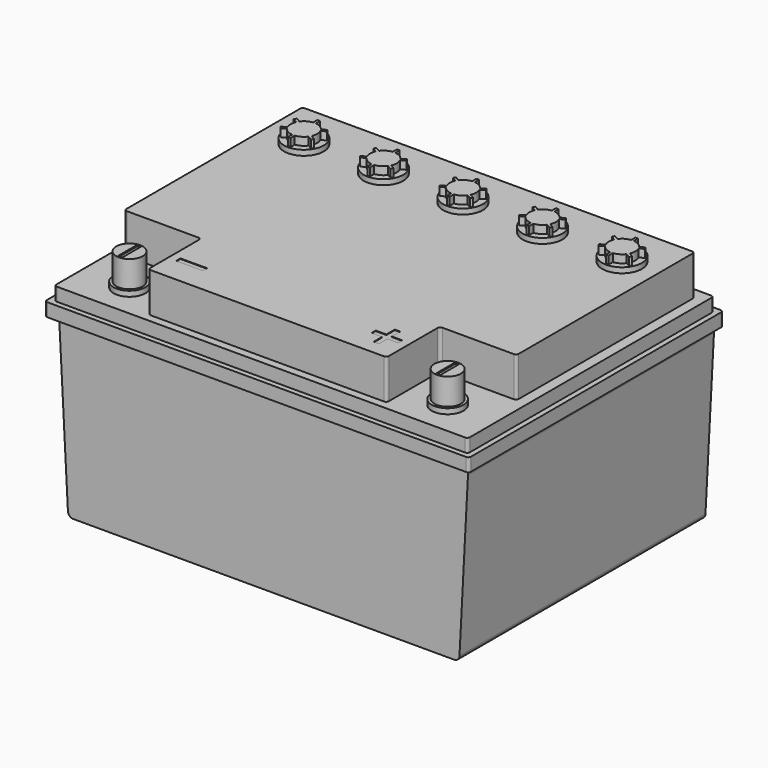
from build123d import *

# Parameters (mm, degrees)
F0_W      = 160
F0_H      = 120
F1_DEPTH  = 5
F2_W      = 156
F2_H      = 116
F3_DEPTH  = 5
F5_DEPTH  = 15
F6_R      = 6
F7_DEPTH  = 2
F8_R      = 5
F9_DEPTH  = 10
F10_R     = 7.5
F11_DEPTH = 2
F13_DEPTH = 3
F14_W     = 1.6
F14_H     = 9.2
F15_DEPTH = 0.5
F16_R     = 1
F17_W     = 10
F17_H     = 1
F18_DEPTH = 0.2
F20_DEPTH = 116


# Not quite as in the source:
# - a feature names something its author has since deleted; it is built from what else it names


with BuildPart() as f1:
    # F0 (on Top) → F1 (new body)
    with BuildSketch(Plane.XY):
        Rectangle(F0_W, F0_H)
    extrude(amount=F1_DEPTH)

    # F2 (on face) → F3 (join)
    with BuildSketch(Plane.XY.offset(5)):
        Rectangle(F2_W, F2_H)
    extrude(amount=F3_DEPTH)

    # F4 (on face) → F5 (join)
    with BuildSketch(Plane.XY.offset(10)):
        Polygon((74, 54), (-74, 54), (-74, -30), (-45, -30), (-45, -55), (45, -55), (45, -30), (74, -30), align=None)
    extrude(amount=F5_DEPTH)

    # F6 (on face) → F7 (join)
    with BuildSketch(Plane.XY.offset(10)):
        with Locations((-60, -45)):
            Circle(F6_R)
        with Locations((60, -45)):
            Circle(F6_R)
    extrude(amount=F7_DEPTH)

    # F8 (on face) → F9 (join)
    with BuildSketch(Plane.XY.offset(12)):
        with Locations((-60, -45)):
            Circle(F8_R)
        with Locations((60, -45)):
            Circle(F8_R)
    extrude(amount=F9_DEPTH)

    # F10 (on face) → F11 (join)
    with BuildSketch(Plane.XY.offset(25)):
        with Locations((-59, 36)):
            Circle(F10_R)
        with Locations((-29, 36)):
            Circle(F10_R)
        with Locations((1, 36)):
            Circle(F10_R)
        with Locations((31, 36)):
            Circle(F10_R)
        with Locations((61, 36)):
            Circle(F10_R)
    extrude(amount=F11_DEPTH)

    # F12 (on face) → F13 (join)
    with BuildSketch(Plane.XY.offset(27)):
        with BuildLine():
            Line((-65.2904727925, 39.0544558909), (-63.5584219849, 38.0544558909))
            ThreePointArc((-63.5584219849, 38.0544558909), (-64, 36), (-63.5584219849, 33.9455441091))
            Line((-63.5584219849, 33.9455441091), (-65.2904727925, 32.9455441091))
            Line((-65.2904727925, 32.9455441091), (-64.7904727925, 32.0795187053))
            Line((-64.7904727925, 32.0795187053), (-63.0584219849, 33.0795187053))
            ThreePointArc((-63.0584219849, 33.0795187053), (-61.5, 31.6698729811), (-59.5, 31.0250628145))
            Line((-59.5, 31.0250628145), (-59.5, 29.0250628145))
            Line((-59.5, 29.0250628145), (-58.5, 29.0250628145))
            Line((-58.5, 29.0250628145), (-58.5, 31.0250628145))
            ThreePointArc((-58.5, 31.0250628145), (-56.5, 31.6698729811), (-54.9415780151, 33.0795187053))
            Line((-54.9415780151, 33.0795187053), (-53.2095272075, 32.0795187053))
            Line((-53.2095272075, 32.0795187053), (-52.7095272075, 32.9455441091))
            Line((-52.7095272075, 32.9455441091), (-54.4415780151, 33.9455441091))
            ThreePointArc((-54.4415780151, 33.9455441091), (-54, 36), (-54.4415780151, 38.0544558909))
            Line((-54.4415780151, 38.0544558909), (-52.7095272075, 39.0544558909))
            Line((-52.7095272075, 39.0544558909), (-53.2095272075, 39.9204812947))
            Line((-53.2095272075, 39.9204812947), (-54.9415780151, 38.9204812947))
            ThreePointArc((-54.9415780151, 38.9204812947), (-56.5, 40.3301270189), (-58.5, 40.9749371855))
            Line((-58.5, 40.9749371855), (-58.5, 42.9749371855))
            Line((-58.5, 42.9749371855), (-59.5, 42.9749371855))
            Line((-59.5, 42.9749371855), (-59.5, 40.9749371855))
            ThreePointArc((-59.5, 40.9749371855), (-61.5, 40.3301270189), (-63.0584219849, 38.9204812947))
            Line((-63.0584219849, 38.9204812947), (-64.7904727925, 39.9204812947))
            Line((-64.7904727925, 39.9204812947), (-65.2904727925, 39.0544558909))
        make_face()
        with BuildLine():
            Line((-28.5, 29.0250628145), (-28.5, 31.0250628145))
            ThreePointArc((-28.5, 31.0250628145), (-26.5, 31.6698729811), (-24.9415780151, 33.0795187053))
            Line((-24.9415780151, 33.0795187053), (-23.2095272075, 32.0795187053))
            Line((-23.2095272075, 32.0795187053), (-22.7095272075, 32.9455441091))
            Line((-22.7095272075, 32.9455441091), (-24.4415780151, 33.9455441091))
            ThreePointArc((-24.4415780151, 33.9455441091), (-24, 36), (-24.4415780151, 38.0544558909))
            Line((-24.4415780151, 38.0544558909), (-22.7095272075, 39.0544558909))
            Line((-22.7095272075, 39.0544558909), (-23.2095272075, 39.9204812947))
            Line((-23.2095272075, 39.9204812947), (-24.9415780151, 38.9204812947))
            ThreePointArc((-24.9415780151, 38.9204812947), (-26.5, 40.3301270189), (-28.5, 40.9749371855))
            Line((-28.5, 40.9749371855), (-28.5, 42.9749371855))
            Line((-28.5, 42.9749371855), (-29.5, 42.9749371855))
            Line((-29.5, 42.9749371855), (-29.5, 40.9749371855))
            ThreePointArc((-29.5, 40.9749371855), (-31.5, 40.3301270189), (-33.0584219849, 38.9204812947))
            Line((-33.0584219849, 38.9204812947), (-34.7904727925, 39.9204812947))
            Line((-34.7904727925, 39.9204812947), (-35.2904727925, 39.0544558909))
            Line((-35.2904727925, 39.0544558909), (-33.5584219849, 38.0544558909))
            ThreePointArc((-33.5584219849, 38.0544558909), (-34, 36), (-33.5584219849, 33.9455441091))
            Line((-33.5584219849, 33.9455441091), (-35.2904727925, 32.9455441091))
            Line((-35.2904727925, 32.9455441091), (-34.7904727925, 32.0795187053))
            Line((-34.7904727925, 32.0795187053), (-33.0584219849, 33.0795187053))
            ThreePointArc((-33.0584219849, 33.0795187053), (-31.5, 31.6698729811), (-29.5, 31.0250628145))
            Line((-29.5, 31.0250628145), (-29.5, 29.0250628145))
            Line((-29.5, 29.0250628145), (-28.5, 29.0250628145))
        make_face()
        with BuildLine():
            Line((1.5, 29.0250628145), (1.5, 31.0250628145))
            ThreePointArc((1.5, 31.0250628145), (3.5, 31.6698729811), (5.0584219849, 33.0795187053))
            Line((5.0584219849, 33.0795187053), (6.7904727925, 32.0795187053))
            Line((6.7904727925, 32.0795187053), (7.2904727925, 32.9455441091))
            Line((7.2904727925, 32.9455441091), (5.5584219849, 33.9455441091))
            ThreePointArc((5.5584219849, 33.9455441091), (6, 36), (5.5584219849, 38.0544558909))
            Line((5.5584219849, 38.0544558909), (7.2904727925, 39.0544558909))
            Line((7.2904727925, 39.0544558909), (6.7904727925, 39.9204812947))
            Line((6.7904727925, 39.9204812947), (5.0584219849, 38.9204812947))
            ThreePointArc((5.0584219849, 38.9204812947), (3.5, 40.3301270189), (1.5, 40.9749371855))
            Line((1.5, 40.9749371855), (1.5, 42.9749371855))
            Line((1.5, 42.9749371855), (0.5, 42.9749371855))
            Line((0.5, 42.9749371855), (0.5, 40.9749371855))
            ThreePointArc((0.5, 40.9749371855), (-1.5, 40.3301270189), (-3.0584219849, 38.9204812947))
            Line((-3.0584219849, 38.9204812947), (-4.7904727925, 39.9204812947))
            Line((-4.7904727925, 39.9204812947), (-5.2904727925, 39.0544558909))
            Line((-5.2904727925, 39.0544558909), (-3.5584219849, 38.0544558909))
            ThreePointArc((-3.5584219849, 38.0544558909), (-4, 36), (-3.5584219849, 33.9455441091))
            Line((-3.5584219849, 33.9455441091), (-5.2904727925, 32.9455441091))
            Line((-5.2904727925, 32.9455441091), (-4.7904727925, 32.0795187053))
            Line((-4.7904727925, 32.0795187053), (-3.0584219849, 33.0795187053))
            ThreePointArc((-3.0584219849, 33.0795187053), (-1.5, 31.6698729811), (0.5, 31.0250628145))
            Line((0.5, 31.0250628145), (0.5, 29.0250628145))
            Line((0.5, 29.0250628145), (1.5, 29.0250628145))
        make_face()
        with BuildLine():
            Line((31.5, 29.0250628145), (31.5, 31.0250628145))
            ThreePointArc((31.5, 31.0250628145), (33.5, 31.6698729811), (35.0584219849, 33.0795187053))
            Line((35.0584219849, 33.0795187053), (36.7904727925, 32.0795187053))
            Line((36.7904727925, 32.0795187053), (37.2904727925, 32.9455441091))
            Line((37.2904727925, 32.9455441091), (35.5584219849, 33.9455441091))
            ThreePointArc((35.5584219849, 33.9455441091), (36, 36), (35.5584219849, 38.0544558909))
            Line((35.5584219849, 38.0544558909), (37.2904727925, 39.0544558909))
            Line((37.2904727925, 39.0544558909), (36.7904727925, 39.9204812947))
            Line((36.7904727925, 39.9204812947), (35.0584219849, 38.9204812947))
            ThreePointArc((35.0584219849, 38.9204812947), (33.5, 40.3301270189), (31.5, 40.9749371855))
            Line((31.5, 40.9749371855), (31.5, 42.9749371855))
            Line((31.5, 42.9749371855), (30.5, 42.9749371855))
            Line((30.5, 42.9749371855), (30.5, 40.9749371855))
            ThreePointArc((30.5, 40.9749371855), (28.5, 40.3301270189), (26.9415780151, 38.9204812947))
            Line((26.9415780151, 38.9204812947), (25.2095272075, 39.9204812947))
            Line((25.2095272075, 39.9204812947), (24.7095272075, 39.0544558909))
            Line((24.7095272075, 39.0544558909), (26.4415780151, 38.0544558909))
            ThreePointArc((26.4415780151, 38.0544558909), (26, 36), (26.4415780151, 33.9455441091))
            Line((26.4415780151, 33.9455441091), (24.7095272075, 32.9455441091))
            Line((24.7095272075, 32.9455441091), (25.2095272075, 32.0795187053))
            Line((25.2095272075, 32.0795187053), (26.9415780151, 33.0795187053))
            ThreePointArc((26.9415780151, 33.0795187053), (28.5, 31.6698729811), (30.5, 31.0250628145))
            Line((30.5, 31.0250628145), (30.5, 29.0250628145))
            Line((30.5, 29.0250628145), (31.5, 29.0250628145))
        make_face()
        with BuildLine():
            Line((61.5, 29.0250628145), (61.5, 31.0250628145))
            ThreePointArc((61.5, 31.0250628145), (63.5, 31.6698729811), (65.0584219849, 33.0795187053))
            Line((65.0584219849, 33.0795187053), (66.7904727925, 32.0795187053))
            Line((66.7904727925, 32.0795187053), (67.2904727925, 32.9455441091))
            Line((67.2904727925, 32.9455441091), (65.5584219849, 33.9455441091))
            ThreePointArc((65.5584219849, 33.9455441091), (66, 36), (65.5584219849, 38.0544558909))
            Line((65.5584219849, 38.0544558909), (67.2904727925, 39.0544558909))
            Line((67.2904727925, 39.0544558909), (66.7904727925, 39.9204812947))
            Line((66.7904727925, 39.9204812947), (65.0584219849, 38.9204812947))
            ThreePointArc((65.0584219849, 38.9204812947), (63.5, 40.3301270189), (61.5, 40.9749371855))
            Line((61.5, 40.9749371855), (61.5, 42.9749371855))
            Line((61.5, 42.9749371855), (60.5, 42.9749371855))
            Line((60.5, 42.9749371855), (60.5, 40.9749371855))
            ThreePointArc((60.5, 40.9749371855), (58.5, 40.3301270189), (56.9415780151, 38.9204812947))
            Line((56.9415780151, 38.9204812947), (55.2095272075, 39.9204812947))
            Line((55.2095272075, 39.9204812947), (54.7095272075, 39.0544558909))
            Line((54.7095272075, 39.0544558909), (56.4415780151, 38.0544558909))
            ThreePointArc((56.4415780151, 38.0544558909), (56, 36), (56.4415780151, 33.9455441091))
            Line((56.4415780151, 33.9455441091), (54.7095272075, 32.9455441091))
            Line((54.7095272075, 32.9455441091), (55.2095272075, 32.0795187053))
            Line((55.2095272075, 32.0795187053), (56.9415780151, 33.0795187053))
            ThreePointArc((56.9415780151, 33.0795187053), (58.5, 31.6698729811), (60.5, 31.0250628145))
            Line((60.5, 31.0250628145), (60.5, 29.0250628145))
            Line((60.5, 29.0250628145), (61.5, 29.0250628145))
        make_face()
    extrude(amount=F13_DEPTH)

    # F14 (on face) → F15 (cut)
    with BuildSketch(Plane.XY.offset(22)):
        with Locations((-60, -45)):
            Rectangle(F14_W, F14_H)
        with Locations((60, -45)):
            Rectangle(F14_W, F14_H)
    extrude(amount=-F15_DEPTH, mode=Mode.SUBTRACT)

    # F16
    f16_edges = [f1.edges().sort_by_distance(p)[0] for p in [
        (45, -55, 17.5),
        (74, -30, 17.5),
        (45, -30, 17.5),
        (-45, -55, 17.5),
        (-45, -30, 17.5),
        (-74, -30, 17.5),
        (-74, 54, 17.5),
        (74, 54, 17.5),
        (78, -58, 7.5),
        (80, -60, 2.5),
        (78, 58, 7.5),
        (80, 60, 2.5),
        (-78, -58, 7.5),
        (-80, -60, 2.5),
        (-78, 58, 7.5),
        (-80, 60, 2.5),
    ]]
    fillet(f16_edges, radius=F16_R)

    # F17 (on face) → F18 (cut)
    with BuildSketch(Plane.XY.offset(25)):
        with Locations((-36.8366418406, -44.1733795106)):
            Rectangle(F17_W, F17_H)
        with Locations((-36.8366418406, -45.1733795106)):
            Rectangle(F17_W, F17_H)
        Polygon((35.8366418406, -43.6733795106), (31.8366418406, -43.6733795106), (31.8366418406, -45.6733795106), (35.8366418406, -45.6733795106), (35.8366418406, -49.6733795106), (37.8366418406, -49.6733795106), (37.8366418406, -45.6733795106), (41.8366418406, -45.6733795106), (41.8366418406, -43.6733795106), (37.8366418406, -43.6733795106), (37.8366418406, -39.6733795106), (35.8366418406, -39.6733795106), align=None)
    extrude(amount=-F18_DEPTH, mode=Mode.SUBTRACT)

    # F19 (on face) → F20 (join)
    with BuildSketch(Plane.XZ.offset(58)):
        with BuildLine():
            Line((76.0839202065, 0.0382618782), (-74.0464704084, 0.0382618782))
            ThreePointArc((-74.0464704084, 0.0382618782), (-75.4972191505, -0.5850289704), (-76.043729478, -2.0664100343))
            Line((-76.043729478, -2.0664100343), (-72.8375185198, -63.2445595772))
            ThreePointArc((-72.8375185198, -63.2445595772), (-72.2169686016, -64.5906364067), (-70.8402594503, -65.1398876647))
            Line((-70.8402594503, -65.1398876647), (72.8777092483, -65.1398876647))
            ThreePointArc((72.8777092483, -65.1398876647), (74.2544183997, -64.5906364067), (74.8749683178, -63.2445595772))
            Line((74.8749683178, -63.2445595772), (78.081179276, -2.0664100343))
            ThreePointArc((78.081179276, -2.0664100343), (77.5346689486, -0.5850289704), (76.0839202065, 0.0382618782))
        make_face()
    extrude(amount=-F20_DEPTH)


solid = f1.part
